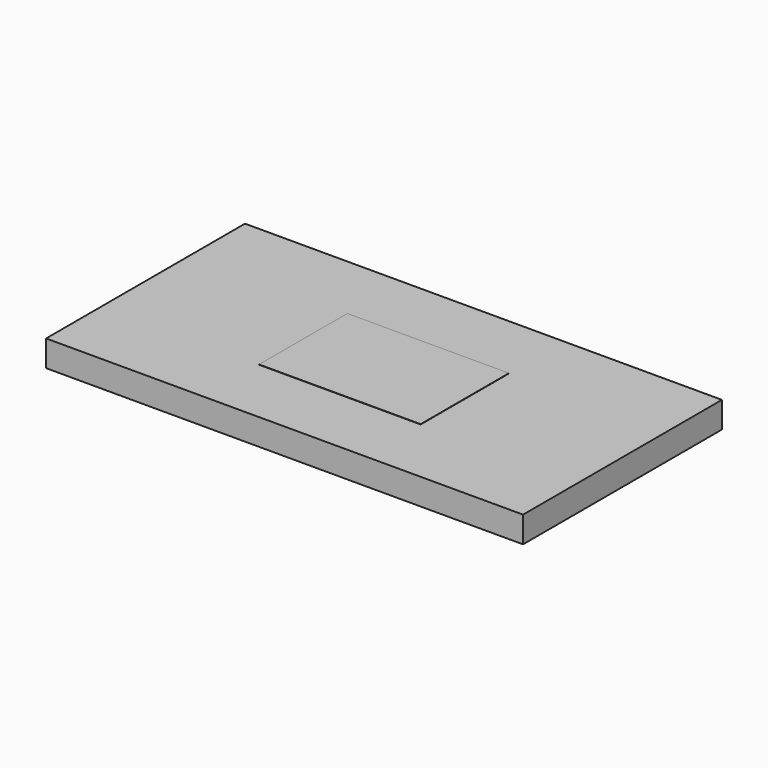
from build123d import *

# Parameters (mm, degrees)
F0_W     = 209.6243202686
F0_H     = 109.2604249716
F0_W_2   = 71
F0_H_2   = 48.5
F1_DEPTH = 11.5
F0_W_3   = 65
F0_H_3   = 42.5
F0_R     = 4.5
F2_DEPTH = 0.125
F3_DEPTH = 3
F4_SIZE  = 2.99999
F5_DEPTH = 0.0625


# Not quite as in the source:
# - a fillet or chamfer is up to 0.001 mm smaller than in the source, because OpenCascade refuses the exact size


with BuildPart() as f1:
    # F0 (on Top) → F1 (new body)
    with BuildSketch(Plane.XY):
        Rectangle(F0_W, F0_H)
        Rectangle(F0_W_2, F0_H_2, mode=Mode.SUBTRACT)
    extrude(amount=-F1_DEPTH)


with BuildPart() as f2:
    # F0 (on Top) → F2 (new body)
    with BuildSketch(Plane.XY):
        Rectangle(F0_W_2, F0_H_2)
        Rectangle(F0_W_3, F0_H_3, mode=Mode.SUBTRACT)
        Rectangle(F0_W_3, F0_H_3)
        with Locations((-22, -10.75)):
            Circle(F0_R, mode=Mode.SUBTRACT)
        with Locations((0, -10.75)):
            Circle(F0_R, mode=Mode.SUBTRACT)
        with Locations((22, -10.75)):
            Circle(F0_R, mode=Mode.SUBTRACT)
        with Locations((-22, 10.75)):
            Circle(F0_R, mode=Mode.SUBTRACT)
        with Locations((0, 10.75)):
            Circle(F0_R, mode=Mode.SUBTRACT)
        with Locations((22, 10.75)):
            Circle(F0_R, mode=Mode.SUBTRACT)
        with Locations((22, -10.75)):
            Circle(F0_R)
        with Locations((0, -10.75)):
            Circle(F0_R)
        with Locations((-22, -10.75)):
            Circle(F0_R)
        with Locations((-22, 10.75)):
            Circle(F0_R)
        with Locations((0, 10.75)):
            Circle(F0_R)
        with Locations((22, 10.75)):
            Circle(F0_R)
    extrude(amount=F2_DEPTH)


with BuildPart() as f3:
    # F0 (on Top) → F3 (new body)
    with BuildSketch(Plane.XY):
        Rectangle(F0_W_2, F0_H_2)
        Rectangle(F0_W_3, F0_H_3, mode=Mode.SUBTRACT)
    extrude(amount=-F3_DEPTH)

    # F4 (size 3 in the source; OpenCascade refuses exactly that, so slightly less here)
    f4_edges = [f3.edges().sort_by_distance(p)[0] for p in [
        (32.5, 0, -3),
        (0, -21.25, -3),
        (0, 21.25, -3),
        (-32.5, 0, -3),
    ]]
    chamfer(f4_edges, length=F4_SIZE)


with BuildPart() as f5:
    # F0 (on Top) → F5 (new body, symmetric)
    with BuildSketch(Plane.XY):
        with Locations((22, -10.75)):
            Circle(F0_R)
    extrude(amount=F5_DEPTH, both=True)


with BuildPart() as f5b:
    # F0 (on Top) → F5, piece 2 (new body, symmetric)
    with BuildSketch(Plane.XY):
        with Locations((22, 10.75)):
            Circle(F0_R)
    extrude(amount=F5_DEPTH, both=True)


with BuildPart() as f5c:
    # F0 (on Top) → F5, piece 3 (new body, symmetric)
    with BuildSketch(Plane.XY):
        with Locations((0, 10.75)):
            Circle(F0_R)
    extrude(amount=F5_DEPTH, both=True)


with BuildPart() as f5d:
    # F0 (on Top) → F5, piece 4 (new body, symmetric)
    with BuildSketch(Plane.XY):
        with Locations((0, -10.75)):
            Circle(F0_R)
    extrude(amount=F5_DEPTH, both=True)


with BuildPart() as f5e:
    # F0 (on Top) → F5, piece 5 (new body, symmetric)
    with BuildSketch(Plane.XY):
        with Locations((-22, 10.75)):
            Circle(F0_R)
    extrude(amount=F5_DEPTH, both=True)


with BuildPart() as f5f:
    # F0 (on Top) → F5, piece 6 (new body, symmetric)
    with BuildSketch(Plane.XY):
        with Locations((-22, -10.75)):
            Circle(F0_R)
    extrude(amount=F5_DEPTH, both=True)


solid = Compound([f1.part, f2.part, f3.part, f5.part, f5b.part, f5c.part, f5d.part, f5e.part, f5f.part])
